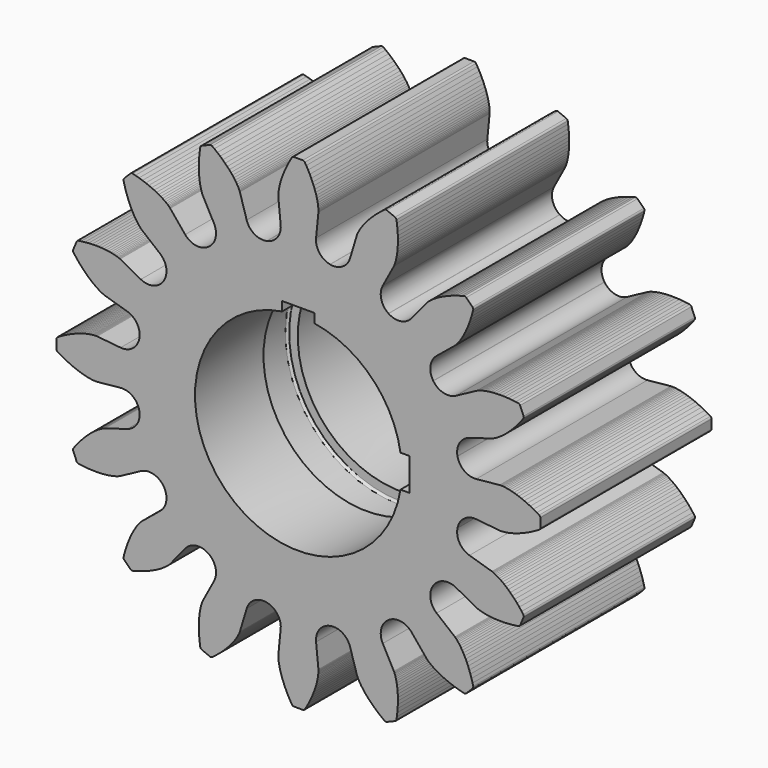
from build123d import *

# Parameters (mm, degrees)
F1_DEPTH = 250


# Not quite as in the source:
# - ends of sketch curves that miss each other by under 0.0002 mm in the source are joined


with BuildPart() as f1:
    # F0 (on Front) → F1 (new body, symmetric)
    with BuildSketch(Plane.XZ):
        with BuildLine():
            ThreePointArc((-371.6747003159, 73.6954086729), (-387.2563589444, 49.0779324218), (-415.3399148314, 41.3240874835))
            Line((-415.3399148314, 41.3240874835), (-470.2256575867, 46.784923388))
            Line((-470.2256575867, 46.784923388), (-471.2844860609, 46.8902713343))
            Line((-471.2844860609, 46.8902713343), (-472.4597318578, 46.9002713343))
            Line((-472.4597318578, 46.9002713343), (-474.0690444775, 46.8465269206))
            Line((-474.0690444775, 46.8465269206), (-476.1124228559, 46.7290391573))
            Line((-476.1124228559, 46.7290391573), (-478.6957490956, 46.5583422005))
            Line((-478.6957490956, 46.5583422005), (-481.6177942115, 46.2074845712))
            Line((-481.6177942115, 46.2074845712), (-485.0797882528, 45.8034166844))
            Line((-485.0797882528, 45.8034166844), (-488.9969184933, 45.1238401788))
            Line((-488.9969184933, 45.1238401788), (-493.252765482, 44.2641030006))
            Line((-493.252765482, 44.2641030006), (-497.963749734, 43.1288550755))
            Line((-497.963749734, 43.1288550755), (-503.1193339008, 41.8239816982))
            Line((-503.1193339008, 41.8239816982), (-508.6347052564, 40.1271813152))
            Line((-508.6347052564, 40.1271813152), (-514.4993296446, 38.1443360289))
            Line((-514.4993296446, 38.1443360289), (-520.8296254522, 35.7800989572))
            Line((-520.8296254522, 35.7800989572), (-527.4032900617, 33.1192817621))
            Line((-527.4032900617, 33.1192817621), (-534.336742924, 30.0665386252))
            Line((-534.336742924, 30.0665386252), (-541.6299829751, 26.6218684827))
            Line((-541.6299829751, 26.6218684827), (-549.1876622686, 22.6688540115))
            Line((-549.1876622686, 22.6688540115), (-556.9992477123, 18.3133773143))
            Line((-556.9992477123, 18.3133773143), (-562.4998031496, 15.0006426899))
            ThreePointArc((-562.4998031496, 15.0006426899), (-564.3868671204, 13.0605402979), (-565.0752713343, 10.4430783145))
            Line((-565.0752713343, 10.4430783145), (-565.0752713343, -10.4430783145))
            ThreePointArc((-565.0752713343, -10.4430783145), (-564.3868671204, -13.0605402979), (-562.4998031027, -15.0006426121))
            Line((-562.4998031027, -15.0006426121), (-556.9992477123, -18.3133773143))
            Line((-556.9992477123, -18.3133773143), (-549.1876622686, -22.6688540115))
            Line((-549.1876622686, -22.6688540115), (-541.6299829751, -26.6218684827))
            Line((-541.6299829751, -26.6218684827), (-534.336742924, -30.0665386252))
            Line((-534.336742924, -30.0665386252), (-527.4032900617, -33.1192817621))
            Line((-527.4032900617, -33.1192817621), (-520.8296254522, -35.7800989572))
            Line((-520.8296254522, -35.7800989572), (-514.4993296446, -38.1443360289))
            Line((-514.4993296446, -38.1443360289), (-508.6347052564, -40.1271813152))
            Line((-508.6347052564, -40.1271813152), (-503.1193339008, -41.8239816982))
            Line((-503.1193339008, -41.8239816982), (-497.963749734, -43.1288550755))
            Line((-497.963749734, -43.1288550755), (-493.252765482, -44.2641030006))
            Line((-493.252765482, -44.2641030006), (-488.9969184933, -45.1238401788))
            Line((-488.9969184933, -45.1238401788), (-485.0797882528, -45.8034166844))
            Line((-485.0797882528, -45.8034166844), (-481.6177942115, -46.2074845712))
            Line((-481.6177942115, -46.2074845712), (-478.6957490956, -46.5583422005))
            Line((-478.6957490956, -46.5583422005), (-476.1124228559, -46.7290391573))
            Line((-476.1124228559, -46.7290391573), (-474.0690444775, -46.8465269206))
            Line((-474.0690444775, -46.8465269206), (-472.4597318578, -46.9002713343))
            Line((-472.4597318578, -46.9002713343), (-471.2844860609, -46.8902713343))
            Line((-471.2844860609, -46.8902713343), (-470.2256575867, -46.784923388))
            Line((-470.2256575867, -46.784923388), (-415.3399148755, -41.3240870398))
            ThreePointArc((-415.3399148755, -41.3240870398), (-387.2563589444, -49.0779324218), (-371.6747003159, -73.6954086729))
            Line((-371.6747003159, -73.6954086729), (-371.5846605661, -74.1480698021))
            ThreePointArc((-371.5846605661, -74.1480698021), (-376.559535795, -102.8544948797), (-399.538090136, -120.7652251933))
            Line((-399.538090136, -120.7652251933), (-452.3356767397, -136.7239348798))
            Line((-452.3356767397, -136.7239348798), (-453.3542211109, -137.0318025112))
            Line((-453.3542211109, -137.0318025112), (-454.4438327304, -137.47231113))
            Line((-454.4438327304, -137.47231113), (-455.910076612, -138.137821877))
            Line((-455.910076612, -138.137821877), (-457.7529516918, -139.028332624))
            Line((-457.7529516918, -139.028332624), (-460.0743115557, -140.1746329006))
            Line((-460.0743115557, -140.1746329006), (-462.6396616301, -141.6170014897))
            Line((-462.6396616301, -141.6170014897), (-465.6834975527, -143.3151585444))
            Line((-465.6834975527, -143.3151585444), (-469.0423909342, -145.442025963))
            Line((-469.0423909342, -145.442025963), (-472.6452734624, -147.864962758))
            Line((-472.6452734624, -147.864962758), (-476.5632145137, -150.716609917))
            Line((-476.5632145137, -150.716609917), (-480.8269993616, -153.89511279))
            Line((-480.8269993616, -153.89511279), (-485.273200681, -157.5733932752))
            Line((-485.273200681, -157.5733932752), (-489.9326058736, -161.6495988508))
            Line((-489.9326058736, -161.6495988508), (-494.8762811236, -166.2563683763))
            Line((-494.8762811236, -166.2563683763), (-499.9313055969, -171.2302745265))
            Line((-499.9313055969, -171.2302745265), (-505.1687465418, -176.703958289))
            Line((-505.1687465418, -176.703958289), (-510.5886039583, -182.6774217919))
            Line((-510.5886039583, -182.6774217919), (-516.0582357949, -189.2217301554))
            Line((-516.0582357949, -189.2217301554), (-521.6084305171, -196.2350297936))
            Line((-521.6084305171, -196.2350297936), (-525.4225526708, -201.400568206))
            ThreePointArc((-525.4225526708, -201.400568206), (-526.4235272395, -203.9151369418), (-526.057870578, -206.5967970892))
            Line((-526.057870578, -206.5967970892), (-518.0650840604, -225.8930910832))
            ThreePointArc((-518.0650840604, -225.8930910832), (-516.4274222611, -228.0478695626), (-513.9415578261, -229.1181424759))
            Line((-513.9415578261, -229.1181424759), (-507.5919780804, -230.0737380294))
            Line((-507.5919780804, -230.0737380294), (-498.7082464354, -231.1083102788))
            Line((-498.7082464354, -231.1083102788), (-490.2131070441, -231.8682208981))
            Line((-490.2131070441, -231.8682208981), (-482.1568142158, -232.259678655))
            Line((-482.1568142158, -232.259678655), (-474.5829048734, -232.4267280272))
            Line((-474.5829048734, -232.4267280272), (-467.4913800809, -232.3693690147))
            Line((-467.4913800809, -232.3693690147), (-460.7381953607, -232.1311406682))
            Line((-460.7381953607, -232.1311406682), (-454.5611864226, -231.7187561183))
            Line((-454.5611864226, -231.7187561183), (-448.8163098532, -231.1757544158))
            Line((-448.8163098532, -231.1757544158), (-443.5538178336, -230.4083432645))
            Line((-443.5538178336, -230.4083432645), (-438.7669961694, -229.6543605022))
            Line((-438.7669961694, -229.6543605022), (-434.506098106, -228.8200117046))
            Line((-434.506098106, -228.8200117046), (-430.6270791658, -227.9488380506))
            Line((-430.6270791658, -227.9488380506), (-427.2739838263, -226.9972994254))
            Line((-427.2739838263, -226.9972994254), (-424.4400989572, -226.2032326027))
            Line((-424.4400989572, -226.2032326027), (-421.9880932113, -225.3723387955))
            Line((-421.9880932113, -225.3723387955), (-420.0552968717, -224.6989167908))
            Line((-420.0552968717, -224.6989167908), (-418.5479197702, -224.1327122792))
            Line((-418.5479197702, -224.1327122792), (-417.4659608427, -223.6737273888))
            Line((-417.4659608427, -223.6737273888), (-416.5280453288, -223.1712023835))
            Line((-416.5280453288, -223.1712023835), (-367.9100031922, -197.1221834433))
            ThreePointArc((-367.9100031922, -197.1221834433), (-338.9969126846, -193.5386902079), (-315.1806367021, -210.3194299305))
            Line((-315.1806367021, -210.3194299305), (-314.924224303, -210.7031772718))
            ThreePointArc((-314.924224303, -210.7031772718), (-308.5349362514, -239.1282583902), (-322.9102125402, -264.4691278049))
            Line((-322.9102125402, -264.4691278049), (-365.5816886572, -299.4178144286))
            Line((-365.5816886572, -299.4178144286), (-366.4048850819, -300.092027027))
            Line((-366.4048850819, -300.092027027), (-367.2429804214, -300.9159810598))
            Line((-367.2429804214, -300.9159810598), (-368.3429325388, -302.0919387104))
            Line((-368.3429325388, -302.0919387104), (-369.7047424984, -303.6199021068))
            Line((-369.7047424984, -303.6199021068), (-371.4107299425, -305.567290913))
            Line((-371.4107299425, -305.567290913), (-373.2288337944, -307.8815833156))
            Line((-373.2288337944, -307.8815833156), (-375.3911151309, -310.6153011279))
            Line((-375.3911151309, -310.6153011279), (-377.6804107257, -313.865662907))
            Line((-377.6804107257, -313.865662907), (-380.0818227282, -317.4829282826))
            Line((-380.0818227282, -317.4829282826), (-382.6102500532, -321.616837625))
            Line((-382.6102500532, -321.616837625), (-385.3331134284, -326.1850712918))
            Line((-385.3331134284, -326.1850712918), (-388.0332506916, -331.28484784))
            Line((-388.0332506916, -331.28484784), (-390.7780836348, -336.8338465631))
            Line((-390.7780836348, -336.8338465631), (-393.5825101085, -342.9818099596))
            Line((-393.5825101085, -342.9818099596), (-396.3493115557, -349.5115737391))
            Line((-396.3493115557, -349.5115737391), (-399.0933879549, -356.5728804001))
            Line((-399.0933879549, -356.5728804001), (-401.8147382422, -364.1657299425))
            Line((-401.8147382422, -364.1657299425), (-404.3636209832, -372.3050202171))
            Line((-404.3636209832, -372.3050202171), (-406.8074579698, -380.9084315812))
            Line((-406.8074579698, -380.9084315812), (-408.3544818046, -387.1403692275))
            ThreePointArc((-408.3544818046, -387.1403692275), (-408.316978103, -389.8465841018), (-406.9529287145, -392.1841843008))
            Line((-406.9529287145, -392.1841843008), (-392.1841838689, -406.9529282826))
            ThreePointArc((-392.1841838689, -406.9529282826), (-389.8465841018, -408.316978103), (-387.140369236, -408.3544817703))
            Line((-387.140369236, -408.3544817703), (-380.9084315812, -406.8074579698))
            Line((-380.9084315812, -406.8074579698), (-372.3050202171, -404.3636209832))
            Line((-372.3050202171, -404.3636209832), (-364.1657299425, -401.8147382422))
            Line((-364.1657299425, -401.8147382422), (-356.5728804001, -399.0933879549))
            Line((-356.5728804001, -399.0933879549), (-349.5115737391, -396.3493115557))
            Line((-349.5115737391, -396.3493115557), (-342.9818099596, -393.5825101085))
            Line((-342.9818099596, -393.5825101085), (-336.8338465631, -390.7780836348))
            Line((-336.8338465631, -390.7780836348), (-331.28484784, -388.0332506916))
            Line((-331.28484784, -388.0332506916), (-326.1850712918, -385.3331134284))
            Line((-326.1850712918, -385.3331134284), (-321.616837625, -382.6102500532))
            Line((-321.616837625, -382.6102500532), (-317.4829282826, -380.0818227282))
            Line((-317.4829282826, -380.0818227282), (-313.865662907, -377.6804107257))
            Line((-313.865662907, -377.6804107257), (-310.6153011279, -375.3911151309))
            Line((-310.6153011279, -375.3911151309), (-307.8815833156, -373.2288337944))
            Line((-307.8815833156, -373.2288337944), (-305.567290913, -371.4107299425))
            Line((-305.567290913, -371.4107299425), (-303.6199021068, -369.7047424984))
            Line((-303.6199021068, -369.7047424984), (-302.0919387104, -368.3429325388))
            Line((-302.0919387104, -368.3429325388), (-300.9159810598, -367.2429804214))
            Line((-300.9159810598, -367.2429804214), (-300.092027027, -366.4048850819))
            Line((-300.092027027, -366.4048850819), (-299.4178144286, -365.5816886572))
            Line((-299.4178144286, -365.5816886572), (-264.4691274739, -322.9102128112))
            ThreePointArc((-264.4691274739, -322.9102128112), (-239.1282583902, -308.5349362514), (-210.7031774657, -314.924224593))
            Line((-210.7031774657, -314.924224593), (-210.3194296659, -315.1806363056))
            ThreePointArc((-210.3194296659, -315.1806363056), (-193.5386902079, -338.9969126846), (-197.1221834078, -367.9100032112))
            Line((-197.1221834078, -367.9100032112), (-223.1712023835, -416.5280453288))
            Line((-223.1712023835, -416.5280453288), (-223.6737273888, -417.4659608427))
            Line((-223.6737273888, -417.4659608427), (-224.1327122792, -418.5479197702))
            Line((-224.1327122792, -418.5479197702), (-224.6989167908, -420.0552968717))
            Line((-224.6989167908, -420.0552968717), (-225.3723387955, -421.9880932113))
            Line((-225.3723387955, -421.9880932113), (-226.2032326027, -424.4400989572))
            Line((-226.2032326027, -424.4400989572), (-226.9972994254, -427.2739838263))
            Line((-226.9972994254, -427.2739838263), (-227.9488380506, -430.6270791658))
            Line((-227.9488380506, -430.6270791658), (-228.8200117046, -434.506098106))
            Line((-228.8200117046, -434.506098106), (-229.6543605022, -438.7669961694))
            Line((-229.6543605022, -438.7669961694), (-230.4083432645, -443.5538178336))
            Line((-230.4083432645, -443.5538178336), (-231.1757544158, -448.8163098532))
            Line((-231.1757544158, -448.8163098532), (-231.7187561183, -454.5611864226))
            Line((-231.7187561183, -454.5611864226), (-232.1311406682, -460.7381953607))
            Line((-232.1311406682, -460.7381953607), (-232.3693690147, -467.4913800809))
            Line((-232.3693690147, -467.4913800809), (-232.4267280272, -474.5829048734))
            Line((-232.4267280272, -474.5829048734), (-232.259678655, -482.1568142158))
            Line((-232.259678655, -482.1568142158), (-231.8682208981, -490.2131070441))
            Line((-231.8682208981, -490.2131070441), (-231.1083102788, -498.7082464354))
            Line((-231.1083102788, -498.7082464354), (-230.0737380294, -507.5919780804))
            Line((-230.0737380294, -507.5919780804), (-229.1181421579, -513.9415577783))
            ThreePointArc((-229.1181421579, -513.9415577783), (-228.0478695626, -516.4274222611), (-225.8930909815, -518.0650838148))
            Line((-225.8930909815, -518.0650838148), (-206.5967971909, -526.0578708236))
            ThreePointArc((-206.5967971909, -526.0578708236), (-203.9151369418, -526.4235272395), (-201.4005682383, -525.4225526271))
            Line((-201.4005682383, -525.4225526271), (-196.2350297936, -521.6084305171))
            Line((-196.2350297936, -521.6084305171), (-189.2217301554, -516.0582357949))
            Line((-189.2217301554, -516.0582357949), (-182.6774217919, -510.5886039583))
            Line((-182.6774217919, -510.5886039583), (-176.703958289, -505.1687465418))
            Line((-176.703958289, -505.1687465418), (-171.2302745265, -499.9313055969))
            Line((-171.2302745265, -499.9313055969), (-166.2563683763, -494.8762811236))
            Line((-166.2563683763, -494.8762811236), (-161.6495988508, -489.9326058736))
            Line((-161.6495988508, -489.9326058736), (-157.5733932752, -485.273200681))
            Line((-157.5733932752, -485.273200681), (-153.89511279, -480.8269993616))
            Line((-153.89511279, -480.8269993616), (-150.716609917, -476.5632145137))
            Line((-150.716609917, -476.5632145137), (-147.864962758, -472.6452734624))
            Line((-147.864962758, -472.6452734624), (-145.442025963, -469.0423909342))
            Line((-145.442025963, -469.0423909342), (-143.3151585444, -465.6834975527))
            Line((-143.3151585444, -465.6834975527), (-141.6170014897, -462.6396616301))
            Line((-141.6170014897, -462.6396616301), (-140.1746329006, -460.0743115557))
            Line((-140.1746329006, -460.0743115557), (-139.028332624, -457.7529516918))
            Line((-139.028332624, -457.7529516918), (-138.137821877, -455.910076612))
            Line((-138.137821877, -455.910076612), (-137.47231113, -454.4438327304))
            Line((-137.47231113, -454.4438327304), (-137.0318025112, -453.3542211109))
            Line((-137.0318025112, -453.3542211109), (-136.7239348798, -452.3356767397))
            Line((-136.7239348798, -452.3356767397), (-120.7652255799, -399.5380900192))
            ThreePointArc((-120.7652255799, -399.5380900192), (-102.8544948797, -376.559535795), (-74.1480698423, -371.5846607676))
            Line((-74.1480698423, -371.5846607676), (-73.6954085976, -371.6746999362))
            ThreePointArc((-73.6954085976, -371.6746999362), (-49.0779324218, -387.2563589444), (-41.3240874835, -415.3399148314))
            Line((-41.3240874835, -415.3399148314), (-46.784923388, -470.2256575867))
            Line((-46.784923388, -470.2256575867), (-46.8902713343, -471.2844860609))
            Line((-46.8902713343, -471.2844860609), (-46.9002713343, -472.4597318578))
            Line((-46.9002713343, -472.4597318578), (-46.8465269206, -474.0690444775))
            Line((-46.8465269206, -474.0690444775), (-46.7290391573, -476.1124228559))
            Line((-46.7290391573, -476.1124228559), (-46.5583422005, -478.6957490956))
            Line((-46.5583422005, -478.6957490956), (-46.2074845712, -481.6177942115))
            Line((-46.2074845712, -481.6177942115), (-45.8034166844, -485.0797882528))
            Line((-45.8034166844, -485.0797882528), (-45.1238401788, -488.9969184933))
            Line((-45.1238401788, -488.9969184933), (-44.2641030006, -493.252765482))
            Line((-44.2641030006, -493.252765482), (-43.1288550755, -497.963749734))
            Line((-43.1288550755, -497.963749734), (-41.8239816982, -503.1193339008))
            Line((-41.8239816982, -503.1193339008), (-40.1271813152, -508.6347052564))
            Line((-40.1271813152, -508.6347052564), (-38.1443360289, -514.4993296446))
            Line((-38.1443360289, -514.4993296446), (-35.7800989572, -520.8296254522))
            Line((-35.7800989572, -520.8296254522), (-33.1192817621, -527.4032900617))
            Line((-33.1192817621, -527.4032900617), (-30.0665386252, -534.336742924))
            Line((-30.0665386252, -534.336742924), (-26.6218684827, -541.6299829751))
            Line((-26.6218684827, -541.6299829751), (-22.6688540115, -549.1876622686))
            Line((-22.6688540115, -549.1876622686), (-18.3133773143, -556.9992477123))
            Line((-18.3133773143, -556.9992477123), (-15.0006426899, -562.4998031496))
            ThreePointArc((-15.0006426899, -562.4998031496), (-13.0605402979, -564.3868671204), (-10.4430783145, -565.0752713343))
            Line((-10.4430783145, -565.0752713343), (10.4430783145, -565.0752713343))
            ThreePointArc((10.4430783145, -565.0752713343), (13.0605402979, -564.3868671204), (15.0006426121, -562.4998031027))
            Line((15.0006426121, -562.4998031027), (18.3133773143, -556.9992477123))
            Line((18.3133773143, -556.9992477123), (22.6688540115, -549.1876622686))
            Line((22.6688540115, -549.1876622686), (26.6218684827, -541.6299829751))
            Line((26.6218684827, -541.6299829751), (30.0665386252, -534.336742924))
            Line((30.0665386252, -534.336742924), (33.1192817621, -527.4032900617))
            Line((33.1192817621, -527.4032900617), (35.7800989572, -520.8296254522))
            Line((35.7800989572, -520.8296254522), (38.1443360289, -514.4993296446))
            Line((38.1443360289, -514.4993296446), (40.1271813152, -508.6347052564))
            Line((40.1271813152, -508.6347052564), (41.8239816982, -503.1193339008))
            Line((41.8239816982, -503.1193339008), (43.1288550755, -497.963749734))
            Line((43.1288550755, -497.963749734), (44.2641030006, -493.252765482))
            Line((44.2641030006, -493.252765482), (45.1238401788, -488.9969184933))
            Line((45.1238401788, -488.9969184933), (45.8034166844, -485.0797882528))
            Line((45.8034166844, -485.0797882528), (46.2074845712, -481.6177942115))
            Line((46.2074845712, -481.6177942115), (46.5583422005, -478.6957490956))
            Line((46.5583422005, -478.6957490956), (46.7290391573, -476.1124228559))
            Line((46.7290391573, -476.1124228559), (46.8465269206, -474.0690444775))
            Line((46.8465269206, -474.0690444775), (46.9002713343, -472.4597318578))
            Line((46.9002713343, -472.4597318578), (46.8902713343, -471.2844860609))
            Line((46.8902713343, -471.2844860609), (46.784923388, -470.2256575867))
            Line((46.784923388, -470.2256575867), (41.3240870398, -415.3399148755))
            ThreePointArc((41.3240870398, -415.3399148755), (49.0779324218, -387.2563589444), (73.6954086729, -371.6747003159))
            Line((73.6954086729, -371.6747003159), (74.1480698021, -371.5846605661))
            ThreePointArc((74.1480698021, -371.5846605661), (102.8544948797, -376.559535795), (120.7652251933, -399.538090136))
            Line((120.7652251933, -399.538090136), (136.7239348798, -452.3356767397))
            Line((136.7239348798, -452.3356767397), (137.0318025112, -453.3542211109))
            Line((137.0318025112, -453.3542211109), (137.47231113, -454.4438327304))
            Line((137.47231113, -454.4438327304), (138.137821877, -455.910076612))
            Line((138.137821877, -455.910076612), (139.028332624, -457.7529516918))
            Line((139.028332624, -457.7529516918), (140.1746329006, -460.0743115557))
            Line((140.1746329006, -460.0743115557), (141.6170014897, -462.6396616301))
            Line((141.6170014897, -462.6396616301), (143.3151585444, -465.6834975527))
            Line((143.3151585444, -465.6834975527), (145.442025963, -469.0423909342))
            Line((145.442025963, -469.0423909342), (147.864962758, -472.6452734624))
            Line((147.864962758, -472.6452734624), (150.716609917, -476.5632145137))
            Line((150.716609917, -476.5632145137), (153.89511279, -480.8269993616))
            Line((153.89511279, -480.8269993616), (157.5733932752, -485.273200681))
            Line((157.5733932752, -485.273200681), (161.6495988508, -489.9326058736))
            Line((161.6495988508, -489.9326058736), (166.2563683763, -494.8762811236))
            Line((166.2563683763, -494.8762811236), (171.2302745265, -499.9313055969))
            Line((171.2302745265, -499.9313055969), (176.703958289, -505.1687465418))
            Line((176.703958289, -505.1687465418), (182.6774217919, -510.5886039583))
            Line((182.6774217919, -510.5886039583), (189.2217301554, -516.0582357949))
            Line((189.2217301554, -516.0582357949), (196.2350297936, -521.6084305171))
            Line((196.2350297936, -521.6084305171), (201.400568206, -525.4225526708))
            ThreePointArc((201.400568206, -525.4225526708), (203.9151369418, -526.4235272395), (206.5967970892, -526.057870578))
            Line((206.5967970892, -526.057870578), (225.8930910832, -518.0650840604))
            ThreePointArc((225.8930910832, -518.0650840604), (228.0478695626, -516.4274222611), (229.1181424759, -513.9415578261))
            Line((229.1181424759, -513.9415578261), (230.0737380294, -507.5919780804))
            Line((230.0737380294, -507.5919780804), (231.1083102788, -498.7082464354))
            Line((231.1083102788, -498.7082464354), (231.8682208981, -490.2131070441))
            Line((231.8682208981, -490.2131070441), (232.259678655, -482.1568142158))
            Line((232.259678655, -482.1568142158), (232.4267280272, -474.5829048734))
            Line((232.4267280272, -474.5829048734), (232.3693690147, -467.4913800809))
            Line((232.3693690147, -467.4913800809), (232.1311406682, -460.7381953607))
            Line((232.1311406682, -460.7381953607), (231.7187561183, -454.5611864226))
            Line((231.7187561183, -454.5611864226), (231.1757544158, -448.8163098532))
            Line((231.1757544158, -448.8163098532), (230.4083432645, -443.5538178336))
            Line((230.4083432645, -443.5538178336), (229.6543605022, -438.7669961694))
            Line((229.6543605022, -438.7669961694), (228.8200117046, -434.506098106))
            Line((228.8200117046, -434.506098106), (227.9488380506, -430.6270791658))
            Line((227.9488380506, -430.6270791658), (226.9972994254, -427.2739838263))
            Line((226.9972994254, -427.2739838263), (226.2032326027, -424.4400989572))
            Line((226.2032326027, -424.4400989572), (225.3723387955, -421.9880932113))
            Line((225.3723387955, -421.9880932113), (224.6989167908, -420.0552968717))
            Line((224.6989167908, -420.0552968717), (224.1327122792, -418.5479197702))
            Line((224.1327122792, -418.5479197702), (223.6737273888, -417.4659608427))
            Line((223.6737273888, -417.4659608427), (223.1712023835, -416.5280453288))
            Line((223.1712023835, -416.5280453288), (197.1221834433, -367.9100031922))
            ThreePointArc((197.1221834433, -367.9100031922), (193.5386902079, -338.9969126846), (210.3194299305, -315.1806367021))
            Line((210.3194299305, -315.1806367021), (210.7031772718, -314.924224303))
            ThreePointArc((210.7031772718, -314.924224303), (239.1282583902, -308.5349362514), (264.4691278049, -322.9102125402))
            Line((264.4691278049, -322.9102125402), (299.4178144286, -365.5816886572))
            Line((299.4178144286, -365.5816886572), (300.092027027, -366.4048850819))
            Line((300.092027027, -366.4048850819), (300.9159810598, -367.2429804214))
            Line((300.9159810598, -367.2429804214), (302.0919387104, -368.3429325388))
            Line((302.0919387104, -368.3429325388), (303.6199021068, -369.7047424984))
            Line((303.6199021068, -369.7047424984), (305.567290913, -371.4107299425))
            Line((305.567290913, -371.4107299425), (307.8815833156, -373.2288337944))
            Line((307.8815833156, -373.2288337944), (310.6153011279, -375.3911151309))
            Line((310.6153011279, -375.3911151309), (313.865662907, -377.6804107257))
            Line((313.865662907, -377.6804107257), (317.4829282826, -380.0818227282))
            Line((317.4829282826, -380.0818227282), (321.616837625, -382.6102500532))
            Line((321.616837625, -382.6102500532), (326.1850712918, -385.3331134284))
            Line((326.1850712918, -385.3331134284), (331.28484784, -388.0332506916))
            Line((331.28484784, -388.0332506916), (336.8338465631, -390.7780836348))
            Line((336.8338465631, -390.7780836348), (342.9818099596, -393.5825101085))
            Line((342.9818099596, -393.5825101085), (349.5115737391, -396.3493115557))
            Line((349.5115737391, -396.3493115557), (356.5728804001, -399.0933879549))
            Line((356.5728804001, -399.0933879549), (364.1657299425, -401.8147382422))
            Line((364.1657299425, -401.8147382422), (372.3050202171, -404.3636209832))
            Line((372.3050202171, -404.3636209832), (380.9084315812, -406.8074579698))
            Line((380.9084315812, -406.8074579698), (387.1403692275, -408.3544818046))
            ThreePointArc((387.1403692275, -408.3544818046), (389.8465841018, -408.316978103), (392.1841843008, -406.9529287145))
            Line((392.1841843008, -406.9529287145), (406.9529282826, -392.1841838689))
            ThreePointArc((406.9529282826, -392.1841838689), (408.316978103, -389.8465841018), (408.3544817703, -387.140369236))
            Line((408.3544817703, -387.140369236), (406.8074579698, -380.9084315812))
            Line((406.8074579698, -380.9084315812), (404.3636209832, -372.3050202171))
            Line((404.3636209832, -372.3050202171), (401.8147382422, -364.1657299425))
            Line((401.8147382422, -364.1657299425), (399.0933879549, -356.5728804001))
            Line((399.0933879549, -356.5728804001), (396.3493115557, -349.5115737391))
            Line((396.3493115557, -349.5115737391), (393.5825101085, -342.9818099596))
            Line((393.5825101085, -342.9818099596), (390.7780836348, -336.8338465631))
            Line((390.7780836348, -336.8338465631), (388.0332506916, -331.28484784))
            Line((388.0332506916, -331.28484784), (385.3331134284, -326.1850712918))
            Line((385.3331134284, -326.1850712918), (382.6102500532, -321.616837625))
            Line((382.6102500532, -321.616837625), (380.0818227282, -317.4829282826))
            Line((380.0818227282, -317.4829282826), (377.6804107257, -313.865662907))
            Line((377.6804107257, -313.865662907), (375.3911151309, -310.6153011279))
            Line((375.3911151309, -310.6153011279), (373.2288337944, -307.8815833156))
            Line((373.2288337944, -307.8815833156), (371.4107299425, -305.567290913))
            Line((371.4107299425, -305.567290913), (369.7047424984, -303.6199021068))
            Line((369.7047424984, -303.6199021068), (368.3429325388, -302.0919387104))
            Line((368.3429325388, -302.0919387104), (367.2429804214, -300.9159810598))
            Line((367.2429804214, -300.9159810598), (366.4048850819, -300.092027027))
            Line((366.4048850819, -300.092027027), (365.5816886572, -299.4178144286))
            Line((365.5816886572, -299.4178144286), (322.9102128112, -264.4691274739))
            ThreePointArc((322.9102128112, -264.4691274739), (308.5349362514, -239.1282583902), (314.924224593, -210.7031774657))
            Line((314.924224593, -210.7031774657), (315.1806363056, -210.3194296659))
            ThreePointArc((315.1806363056, -210.3194296659), (338.9969126846, -193.5386902079), (367.9100032112, -197.1221834078))
            Line((367.9100032112, -197.1221834078), (416.5280453288, -223.1712023835))
            Line((416.5280453288, -223.1712023835), (417.4659608427, -223.6737273888))
            Line((417.4659608427, -223.6737273888), (418.5479197702, -224.1327122792))
            Line((418.5479197702, -224.1327122792), (420.0552968717, -224.6989167908))
            Line((420.0552968717, -224.6989167908), (421.9880932113, -225.3723387955))
            Line((421.9880932113, -225.3723387955), (424.4400989572, -226.2032326027))
            Line((424.4400989572, -226.2032326027), (427.2739838263, -226.9972994254))
            Line((427.2739838263, -226.9972994254), (430.6270791658, -227.9488380506))
            Line((430.6270791658, -227.9488380506), (434.506098106, -228.8200117046))
            Line((434.506098106, -228.8200117046), (438.7669961694, -229.6543605022))
            Line((438.7669961694, -229.6543605022), (443.5538178336, -230.4083432645))
            Line((443.5538178336, -230.4083432645), (448.8163098532, -231.1757544158))
            Line((448.8163098532, -231.1757544158), (454.5611864226, -231.7187561183))
            Line((454.5611864226, -231.7187561183), (460.7381953607, -232.1311406682))
            Line((460.7381953607, -232.1311406682), (467.4913800809, -232.3693690147))
            Line((467.4913800809, -232.3693690147), (474.5829048734, -232.4267280272))
            Line((474.5829048734, -232.4267280272), (482.1568142158, -232.259678655))
            Line((482.1568142158, -232.259678655), (490.2131070441, -231.8682208981))
            Line((490.2131070441, -231.8682208981), (498.7082464354, -231.1083102788))
            Line((498.7082464354, -231.1083102788), (507.5919780804, -230.0737380294))
            Line((507.5919780804, -230.0737380294), (513.9415577783, -229.1181421579))
            ThreePointArc((513.9415577783, -229.1181421579), (516.4274222611, -228.0478695626), (518.0650838148, -225.8930909815))
            Line((518.0650838148, -225.8930909815), (526.0578708236, -206.5967971909))
            ThreePointArc((526.0578708236, -206.5967971909), (526.4235272395, -203.9151369418), (525.4225526271, -201.4005682383))
            Line((525.4225526271, -201.4005682383), (521.6084305171, -196.2350297936))
            Line((521.6084305171, -196.2350297936), (516.0582357949, -189.2217301554))
            Line((516.0582357949, -189.2217301554), (510.5886039583, -182.6774217919))
            Line((510.5886039583, -182.6774217919), (505.1687465418, -176.703958289))
            Line((505.1687465418, -176.703958289), (499.9313055969, -171.2302745265))
            Line((499.9313055969, -171.2302745265), (494.8762811236, -166.2563683763))
            Line((494.8762811236, -166.2563683763), (489.9326058736, -161.6495988508))
            Line((489.9326058736, -161.6495988508), (485.273200681, -157.5733932752))
            Line((485.273200681, -157.5733932752), (480.8269993616, -153.89511279))
            Line((480.8269993616, -153.89511279), (476.5632145137, -150.716609917))
            Line((476.5632145137, -150.716609917), (472.6452734624, -147.864962758))
            Line((472.6452734624, -147.864962758), (469.0423909342, -145.442025963))
            Line((469.0423909342, -145.442025963), (465.6834975527, -143.3151585444))
            Line((465.6834975527, -143.3151585444), (462.6396616301, -141.6170014897))
            Line((462.6396616301, -141.6170014897), (460.0743115557, -140.1746329006))
            Line((460.0743115557, -140.1746329006), (457.7529516918, -139.028332624))
            Line((457.7529516918, -139.028332624), (455.910076612, -138.137821877))
            Line((455.910076612, -138.137821877), (454.4438327304, -137.47231113))
            Line((454.4438327304, -137.47231113), (453.3542211109, -137.0318025112))
            Line((453.3542211109, -137.0318025112), (452.3356767397, -136.7239348798))
            Line((452.3356767397, -136.7239348798), (399.5380900192, -120.7652255799))
            ThreePointArc((399.5380900192, -120.7652255799), (376.559535795, -102.8544948797), (371.5846607676, -74.1480698423))
            Line((371.5846607676, -74.1480698423), (371.6746999362, -73.6954085976))
            ThreePointArc((371.6746999362, -73.6954085976), (387.2563589444, -49.0779324218), (415.3399148314, -41.3240874835))
            Line((415.3399148314, -41.3240874835), (470.2256575867, -46.784923388))
            Line((470.2256575867, -46.784923388), (471.2844860609, -46.8902713343))
            Line((471.2844860609, -46.8902713343), (472.4597318578, -46.9002713343))
            Line((472.4597318578, -46.9002713343), (474.0690444775, -46.8465269206))
            Line((474.0690444775, -46.8465269206), (476.1124228559, -46.7290391573))
            Line((476.1124228559, -46.7290391573), (478.6957490956, -46.5583422005))
            Line((478.6957490956, -46.5583422005), (481.6177942115, -46.2074845712))
            Line((481.6177942115, -46.2074845712), (485.0797882528, -45.8034166844))
            Line((485.0797882528, -45.8034166844), (488.9969184933, -45.1238401788))
            Line((488.9969184933, -45.1238401788), (493.252765482, -44.2641030006))
            Line((493.252765482, -44.2641030006), (497.963749734, -43.1288550755))
            Line((497.963749734, -43.1288550755), (503.1193339008, -41.8239816982))
            Line((503.1193339008, -41.8239816982), (508.6347052564, -40.1271813152))
            Line((508.6347052564, -40.1271813152), (514.4993296446, -38.1443360289))
            Line((514.4993296446, -38.1443360289), (520.8296254522, -35.7800989572))
            Line((520.8296254522, -35.7800989572), (527.4032900617, -33.1192817621))
            Line((527.4032900617, -33.1192817621), (534.336742924, -30.0665386252))
            Line((534.336742924, -30.0665386252), (541.6299829751, -26.6218684827))
            Line((541.6299829751, -26.6218684827), (549.1876622686, -22.6688540115))
            Line((549.1876622686, -22.6688540115), (556.9992477123, -18.3133773143))
            Line((556.9992477123, -18.3133773143), (562.4998031496, -15.0006426899))
            ThreePointArc((562.4998031496, -15.0006426899), (564.3868671204, -13.0605402979), (565.0752713343, -10.4430783145))
            Line((565.0752713343, -10.4430783145), (565.0752713343, 10.4430783145))
            ThreePointArc((565.0752713343, 10.4430783145), (564.3868671204, 13.0605402979), (562.4998031027, 15.0006426121))
            Line((562.4998031027, 15.0006426121), (556.9992477123, 18.3133773143))
            Line((556.9992477123, 18.3133773143), (549.1876622686, 22.6688540115))
            Line((549.1876622686, 22.6688540115), (541.6299829751, 26.6218684827))
            Line((541.6299829751, 26.6218684827), (534.336742924, 30.0665386252))
            Line((534.336742924, 30.0665386252), (527.4032900617, 33.1192817621))
            Line((527.4032900617, 33.1192817621), (520.8296254522, 35.7800989572))
            Line((520.8296254522, 35.7800989572), (514.4993296446, 38.1443360289))
            Line((514.4993296446, 38.1443360289), (508.6347052564, 40.1271813152))
            Line((508.6347052564, 40.1271813152), (503.1193339008, 41.8239816982))
            Line((503.1193339008, 41.8239816982), (497.963749734, 43.1288550755))
            Line((497.963749734, 43.1288550755), (493.252765482, 44.2641030006))
            Line((493.252765482, 44.2641030006), (488.9969184933, 45.1238401788))
            Line((488.9969184933, 45.1238401788), (485.0797882528, 45.8034166844))
            Line((485.0797882528, 45.8034166844), (481.6177942115, 46.2074845712))
            Line((481.6177942115, 46.2074845712), (478.6957490956, 46.5583422005))
            Line((478.6957490956, 46.5583422005), (476.1124228559, 46.7290391573))
            Line((476.1124228559, 46.7290391573), (474.0690444775, 46.8465269206))
            Line((474.0690444775, 46.8465269206), (472.4597318578, 46.9002713343))
            Line((472.4597318578, 46.9002713343), (471.2844860609, 46.8902713343))
            Line((471.2844860609, 46.8902713343), (470.2256575867, 46.784923388))
            Line((470.2256575867, 46.784923388), (415.3399148755, 41.3240870398))
            ThreePointArc((415.3399148755, 41.3240870398), (387.2563589444, 49.0779324218), (371.6747003159, 73.6954086729))
            Line((371.6747003159, 73.6954086729), (371.5846605661, 74.1480698021))
            ThreePointArc((371.5846605661, 74.1480698021), (376.559535795, 102.8544948797), (399.538090136, 120.7652251933))
            Line((399.538090136, 120.7652251933), (452.3356767397, 136.7239348798))
            Line((452.3356767397, 136.7239348798), (453.3542211109, 137.0318025112))
            Line((453.3542211109, 137.0318025112), (454.4438327304, 137.47231113))
            Line((454.4438327304, 137.47231113), (455.910076612, 138.137821877))
            Line((455.910076612, 138.137821877), (457.7529516918, 139.028332624))
            Line((457.7529516918, 139.028332624), (460.0743115557, 140.1746329006))
            Line((460.0743115557, 140.1746329006), (462.6396616301, 141.6170014897))
            Line((462.6396616301, 141.6170014897), (465.6834975527, 143.3151585444))
            Line((465.6834975527, 143.3151585444), (469.0423909342, 145.442025963))
            Line((469.0423909342, 145.442025963), (472.6452734624, 147.864962758))
            Line((472.6452734624, 147.864962758), (476.5632145137, 150.716609917))
            Line((476.5632145137, 150.716609917), (480.8269993616, 153.89511279))
            Line((480.8269993616, 153.89511279), (485.273200681, 157.5733932752))
            Line((485.273200681, 157.5733932752), (489.9326058736, 161.6495988508))
            Line((489.9326058736, 161.6495988508), (494.8762811236, 166.2563683763))
            Line((494.8762811236, 166.2563683763), (499.9313055969, 171.2302745265))
            Line((499.9313055969, 171.2302745265), (505.1687465418, 176.703958289))
            Line((505.1687465418, 176.703958289), (510.5886039583, 182.6774217919))
            Line((510.5886039583, 182.6774217919), (516.0582357949, 189.2217301554))
            Line((516.0582357949, 189.2217301554), (521.6084305171, 196.2350297936))
            Line((521.6084305171, 196.2350297936), (525.4225526708, 201.400568206))
            ThreePointArc((525.4225526708, 201.400568206), (526.4235272395, 203.9151369418), (526.057870578, 206.5967970892))
            Line((526.057870578, 206.5967970892), (518.0650840604, 225.8930910832))
            ThreePointArc((518.0650840604, 225.8930910832), (516.4274222611, 228.0478695626), (513.9415578261, 229.1181424759))
            Line((513.9415578261, 229.1181424759), (507.5919780804, 230.0737380294))
            Line((507.5919780804, 230.0737380294), (498.7082464354, 231.1083102788))
            Line((498.7082464354, 231.1083102788), (490.2131070441, 231.8682208981))
            Line((490.2131070441, 231.8682208981), (482.1568142158, 232.259678655))
            Line((482.1568142158, 232.259678655), (474.5829048734, 232.4267280272))
            Line((474.5829048734, 232.4267280272), (467.4913800809, 232.3693690147))
            Line((467.4913800809, 232.3693690147), (460.7381953607, 232.1311406682))
            Line((460.7381953607, 232.1311406682), (454.5611864226, 231.7187561183))
            Line((454.5611864226, 231.7187561183), (448.8163098532, 231.1757544158))
            Line((448.8163098532, 231.1757544158), (443.5538178336, 230.4083432645))
            Line((443.5538178336, 230.4083432645), (438.7669961694, 229.6543605022))
            Line((438.7669961694, 229.6543605022), (434.506098106, 228.8200117046))
            Line((434.506098106, 228.8200117046), (430.6270791658, 227.9488380506))
            Line((430.6270791658, 227.9488380506), (427.2739838263, 226.9972994254))
            Line((427.2739838263, 226.9972994254), (424.4400989572, 226.2032326027))
            Line((424.4400989572, 226.2032326027), (421.9880932113, 225.3723387955))
            Line((421.9880932113, 225.3723387955), (420.0552968717, 224.6989167908))
            Line((420.0552968717, 224.6989167908), (418.5479197702, 224.1327122792))
            Line((418.5479197702, 224.1327122792), (417.4659608427, 223.6737273888))
            Line((417.4659608427, 223.6737273888), (416.5280453288, 223.1712023835))
            Line((416.5280453288, 223.1712023835), (367.9100031922, 197.1221834433))
            ThreePointArc((367.9100031922, 197.1221834433), (338.9969126846, 193.5386902079), (315.1806367021, 210.3194299305))
            Line((315.1806367021, 210.3194299305), (314.924224303, 210.7031772718))
            ThreePointArc((314.924224303, 210.7031772718), (308.5349362514, 239.1282583902), (322.9102125402, 264.4691278049))
            Line((322.9102125402, 264.4691278049), (365.5816886572, 299.4178144286))
            Line((365.5816886572, 299.4178144286), (366.4048850819, 300.092027027))
            Line((366.4048850819, 300.092027027), (367.2429804214, 300.9159810598))
            Line((367.2429804214, 300.9159810598), (368.3429325388, 302.0919387104))
            Line((368.3429325388, 302.0919387104), (369.7047424984, 303.6199021068))
            Line((369.7047424984, 303.6199021068), (371.4107299425, 305.567290913))
            Line((371.4107299425, 305.567290913), (373.2288337944, 307.8815833156))
            Line((373.2288337944, 307.8815833156), (375.3911151309, 310.6153011279))
            Line((375.3911151309, 310.6153011279), (377.6804107257, 313.865662907))
            Line((377.6804107257, 313.865662907), (380.0818227282, 317.4829282826))
            Line((380.0818227282, 317.4829282826), (382.6102500532, 321.616837625))
            Line((382.6102500532, 321.616837625), (385.3331134284, 326.1850712918))
            Line((385.3331134284, 326.1850712918), (388.0332506916, 331.28484784))
            Line((388.0332506916, 331.28484784), (390.7780836348, 336.8338465631))
            Line((390.7780836348, 336.8338465631), (393.5825101085, 342.9818099596))
            Line((393.5825101085, 342.9818099596), (396.3493115557, 349.5115737391))
            Line((396.3493115557, 349.5115737391), (399.0933879549, 356.5728804001))
            Line((399.0933879549, 356.5728804001), (401.8147382422, 364.1657299425))
            Line((401.8147382422, 364.1657299425), (404.3636209832, 372.3050202171))
            Line((404.3636209832, 372.3050202171), (406.8074579698, 380.9084315812))
            Line((406.8074579698, 380.9084315812), (408.3544818046, 387.1403692275))
            ThreePointArc((408.3544818046, 387.1403692275), (408.316978103, 389.8465841018), (406.9529287145, 392.1841843008))
            Line((406.9529287145, 392.1841843008), (392.1841838689, 406.9529282826))
            ThreePointArc((392.1841838689, 406.9529282826), (389.8465841018, 408.316978103), (387.140369236, 408.3544817703))
            Line((387.140369236, 408.3544817703), (380.9084315812, 406.8074579698))
            Line((380.9084315812, 406.8074579698), (372.3050202171, 404.3636209832))
            Line((372.3050202171, 404.3636209832), (364.1657299425, 401.8147382422))
            Line((364.1657299425, 401.8147382422), (356.5728804001, 399.0933879549))
            Line((356.5728804001, 399.0933879549), (349.5115737391, 396.3493115557))
            Line((349.5115737391, 396.3493115557), (342.9818099596, 393.5825101085))
            Line((342.9818099596, 393.5825101085), (336.8338465631, 390.7780836348))
            Line((336.8338465631, 390.7780836348), (331.28484784, 388.0332506916))
            Line((331.28484784, 388.0332506916), (326.1850712918, 385.3331134284))
            Line((326.1850712918, 385.3331134284), (321.616837625, 382.6102500532))
            Line((321.616837625, 382.6102500532), (317.4829282826, 380.0818227282))
            Line((317.4829282826, 380.0818227282), (313.865662907, 377.6804107257))
            Line((313.865662907, 377.6804107257), (310.6153011279, 375.3911151309))
            Line((310.6153011279, 375.3911151309), (307.8815833156, 373.2288337944))
            Line((307.8815833156, 373.2288337944), (305.567290913, 371.4107299425))
            Line((305.567290913, 371.4107299425), (303.6199021068, 369.7047424984))
            Line((303.6199021068, 369.7047424984), (302.0919387104, 368.3429325388))
            Line((302.0919387104, 368.3429325388), (300.9159810598, 367.2429804214))
            Line((300.9159810598, 367.2429804214), (300.092027027, 366.4048850819))
            Line((300.092027027, 366.4048850819), (299.4178144286, 365.5816886572))
            Line((299.4178144286, 365.5816886572), (264.4691274739, 322.9102128112))
            ThreePointArc((264.4691274739, 322.9102128112), (239.1282583902, 308.5349362514), (210.7031774657, 314.924224593))
            Line((210.7031774657, 314.924224593), (210.3194296659, 315.1806363056))
            ThreePointArc((210.3194296659, 315.1806363056), (193.5386902079, 338.9969126846), (197.1221834078, 367.9100032112))
            Line((197.1221834078, 367.9100032112), (223.1712023835, 416.5280453288))
            Line((223.1712023835, 416.5280453288), (223.6737273888, 417.4659608427))
            Line((223.6737273888, 417.4659608427), (224.1327122792, 418.5479197702))
            Line((224.1327122792, 418.5479197702), (224.6989167908, 420.0552968717))
            Line((224.6989167908, 420.0552968717), (225.3723387955, 421.9880932113))
            Line((225.3723387955, 421.9880932113), (226.2032326027, 424.4400989572))
            Line((226.2032326027, 424.4400989572), (226.9972994254, 427.2739838263))
            Line((226.9972994254, 427.2739838263), (227.9488380506, 430.6270791658))
            Line((227.9488380506, 430.6270791658), (228.8200117046, 434.506098106))
            Line((228.8200117046, 434.506098106), (229.6543605022, 438.7669961694))
            Line((229.6543605022, 438.7669961694), (230.4083432645, 443.5538178336))
            Line((230.4083432645, 443.5538178336), (231.1757544158, 448.8163098532))
            Line((231.1757544158, 448.8163098532), (231.7187561183, 454.5611864226))
            Line((231.7187561183, 454.5611864226), (232.1311406682, 460.7381953607))
            Line((232.1311406682, 460.7381953607), (232.3693690147, 467.4913800809))
            Line((232.3693690147, 467.4913800809), (232.4267280272, 474.5829048734))
            Line((232.4267280272, 474.5829048734), (232.259678655, 482.1568142158))
            Line((232.259678655, 482.1568142158), (231.8682208981, 490.2131070441))
            Line((231.8682208981, 490.2131070441), (231.1083102788, 498.7082464354))
            Line((231.1083102788, 498.7082464354), (230.0737380294, 507.5919780804))
            Line((230.0737380294, 507.5919780804), (229.1181421579, 513.9415577783))
            ThreePointArc((229.1181421579, 513.9415577783), (228.0478695626, 516.4274222611), (225.8930909815, 518.0650838148))
            Line((225.8930909815, 518.0650838148), (206.5967971909, 526.0578708236))
            ThreePointArc((206.5967971909, 526.0578708236), (203.9151369418, 526.4235272395), (201.4005682383, 525.4225526271))
            Line((201.4005682383, 525.4225526271), (196.2350297936, 521.6084305171))
            Line((196.2350297936, 521.6084305171), (189.2217301554, 516.0582357949))
            Line((189.2217301554, 516.0582357949), (182.6774217919, 510.5886039583))
            Line((182.6774217919, 510.5886039583), (176.703958289, 505.1687465418))
            Line((176.703958289, 505.1687465418), (171.2302745265, 499.9313055969))
            Line((171.2302745265, 499.9313055969), (166.2563683763, 494.8762811236))
            Line((166.2563683763, 494.8762811236), (161.6495988508, 489.9326058736))
            Line((161.6495988508, 489.9326058736), (157.5733932752, 485.273200681))
            Line((157.5733932752, 485.273200681), (153.89511279, 480.8269993616))
            Line((153.89511279, 480.8269993616), (150.716609917, 476.5632145137))
            Line((150.716609917, 476.5632145137), (147.864962758, 472.6452734624))
            Line((147.864962758, 472.6452734624), (145.442025963, 469.0423909342))
            Line((145.442025963, 469.0423909342), (143.3151585444, 465.6834975527))
            Line((143.3151585444, 465.6834975527), (141.6170014897, 462.6396616301))
            Line((141.6170014897, 462.6396616301), (140.1746329006, 460.0743115557))
            Line((140.1746329006, 460.0743115557), (139.028332624, 457.7529516918))
            Line((139.028332624, 457.7529516918), (138.137821877, 455.910076612))
            Line((138.137821877, 455.910076612), (137.47231113, 454.4438327304))
            Line((137.47231113, 454.4438327304), (137.0318025112, 453.3542211109))
            Line((137.0318025112, 453.3542211109), (136.7239348798, 452.3356767397))
            Line((136.7239348798, 452.3356767397), (120.7652255799, 399.5380900192))
            ThreePointArc((120.7652255799, 399.5380900192), (102.8544948797, 376.559535795), (74.1480698423, 371.5846607676))
            Line((74.1480698423, 371.5846607676), (73.6954085976, 371.6746999362))
            ThreePointArc((73.6954085976, 371.6746999362), (49.0779324218, 387.2563589444), (41.3240874835, 415.3399148314))
            Line((41.3240874835, 415.3399148314), (46.784923388, 470.2256575867))
            Line((46.784923388, 470.2256575867), (46.8902713343, 471.2844860609))
            Line((46.8902713343, 471.2844860609), (46.9002713343, 472.4597318578))
            Line((46.9002713343, 472.4597318578), (46.8465269206, 474.0690444775))
            Line((46.8465269206, 474.0690444775), (46.7290391573, 476.1124228559))
            Line((46.7290391573, 476.1124228559), (46.5583422005, 478.6957490956))
            Line((46.5583422005, 478.6957490956), (46.2074845712, 481.6177942115))
            Line((46.2074845712, 481.6177942115), (45.8034166844, 485.0797882528))
            Line((45.8034166844, 485.0797882528), (45.1238401788, 488.9969184933))
            Line((45.1238401788, 488.9969184933), (44.2641030006, 493.252765482))
            Line((44.2641030006, 493.252765482), (43.1288550755, 497.963749734))
            Line((43.1288550755, 497.963749734), (41.8239816982, 503.1193339008))
            Line((41.8239816982, 503.1193339008), (40.1271813152, 508.6347052564))
            Line((40.1271813152, 508.6347052564), (38.1443360289, 514.4993296446))
            Line((38.1443360289, 514.4993296446), (35.7800989572, 520.8296254522))
            Line((35.7800989572, 520.8296254522), (33.1192817621, 527.4032900617))
            Line((33.1192817621, 527.4032900617), (30.0665386252, 534.336742924))
            Line((30.0665386252, 534.336742924), (26.6218684827, 541.6299829751))
            Line((26.6218684827, 541.6299829751), (22.6688540115, 549.1876622686))
            Line((22.6688540115, 549.1876622686), (18.3133773143, 556.9992477123))
            Line((18.3133773143, 556.9992477123), (15.0006426899, 562.4998031496))
            ThreePointArc((15.0006426899, 562.4998031496), (13.0605402979, 564.3868671204), (10.4430783145, 565.0752713343))
            Line((10.4430783145, 565.0752713343), (-10.4430783145, 565.0752713343))
            ThreePointArc((-10.4430783145, 565.0752713343), (-13.0605402979, 564.3868671204), (-15.0006426121, 562.4998031027))
            Line((-15.0006426121, 562.4998031027), (-18.3133773143, 556.9992477123))
            Line((-18.3133773143, 556.9992477123), (-22.6688540115, 549.1876622686))
            Line((-22.6688540115, 549.1876622686), (-26.6218684827, 541.6299829751))
            Line((-26.6218684827, 541.6299829751), (-30.0665386252, 534.336742924))
            Line((-30.0665386252, 534.336742924), (-33.1192817621, 527.4032900617))
            Line((-33.1192817621, 527.4032900617), (-35.7800989572, 520.8296254522))
            Line((-35.7800989572, 520.8296254522), (-38.1443360289, 514.4993296446))
            Line((-38.1443360289, 514.4993296446), (-40.1271813152, 508.6347052564))
            Line((-40.1271813152, 508.6347052564), (-41.8239816982, 503.1193339008))
            Line((-41.8239816982, 503.1193339008), (-43.1288550755, 497.963749734))
            Line((-43.1288550755, 497.963749734), (-44.2641030006, 493.252765482))
            Line((-44.2641030006, 493.252765482), (-45.1238401788, 488.9969184933))
            Line((-45.1238401788, 488.9969184933), (-45.8034166844, 485.0797882528))
            Line((-45.8034166844, 485.0797882528), (-46.2074845712, 481.6177942115))
            Line((-46.2074845712, 481.6177942115), (-46.5583422005, 478.6957490956))
            Line((-46.5583422005, 478.6957490956), (-46.7290391573, 476.1124228559))
            Line((-46.7290391573, 476.1124228559), (-46.8465269206, 474.0690444775))
            Line((-46.8465269206, 474.0690444775), (-46.9002713343, 472.4597318578))
            Line((-46.9002713343, 472.4597318578), (-46.8902713343, 471.2844860609))
            Line((-46.8902713343, 471.2844860609), (-46.784923388, 470.2256575867))
            Line((-46.784923388, 470.2256575867), (-41.3240870398, 415.3399148755))
            ThreePointArc((-41.3240870398, 415.3399148755), (-49.0779324218, 387.2563589444), (-73.6954086729, 371.6747003159))
            Line((-73.6954086729, 371.6747003159), (-74.1480698021, 371.5846605661))
            ThreePointArc((-74.1480698021, 371.5846605661), (-102.8544948797, 376.559535795), (-120.7652251933, 399.538090136))
            Line((-120.7652251933, 399.538090136), (-136.7239348798, 452.3356767397))
            Line((-136.7239348798, 452.3356767397), (-137.0318025112, 453.3542211109))
            Line((-137.0318025112, 453.3542211109), (-137.47231113, 454.4438327304))
            Line((-137.47231113, 454.4438327304), (-138.137821877, 455.910076612))
            Line((-138.137821877, 455.910076612), (-139.028332624, 457.7529516918))
            Line((-139.028332624, 457.7529516918), (-140.1746329006, 460.0743115557))
            Line((-140.1746329006, 460.0743115557), (-141.6170014897, 462.6396616301))
            Line((-141.6170014897, 462.6396616301), (-143.3151585444, 465.6834975527))
            Line((-143.3151585444, 465.6834975527), (-145.442025963, 469.0423909342))
            Line((-145.442025963, 469.0423909342), (-147.864962758, 472.6452734624))
            Line((-147.864962758, 472.6452734624), (-150.716609917, 476.5632145137))
            Line((-150.716609917, 476.5632145137), (-153.89511279, 480.8269993616))
            Line((-153.89511279, 480.8269993616), (-157.5733932752, 485.273200681))
            Line((-157.5733932752, 485.273200681), (-161.6495988508, 489.9326058736))
            Line((-161.6495988508, 489.9326058736), (-166.2563683763, 494.8762811236))
            Line((-166.2563683763, 494.8762811236), (-171.2302745265, 499.9313055969))
            Line((-171.2302745265, 499.9313055969), (-176.703958289, 505.1687465418))
            Line((-176.703958289, 505.1687465418), (-182.6774217919, 510.5886039583))
            Line((-182.6774217919, 510.5886039583), (-189.2217301554, 516.0582357949))
            Line((-189.2217301554, 516.0582357949), (-196.2350297936, 521.6084305171))
            Line((-196.2350297936, 521.6084305171), (-201.400568206, 525.4225526708))
            ThreePointArc((-201.400568206, 525.4225526708), (-203.9151369418, 526.4235272395), (-206.5967970892, 526.057870578))
            Line((-206.5967970892, 526.057870578), (-225.8930910832, 518.0650840604))
            ThreePointArc((-225.8930910832, 518.0650840604), (-228.0478695626, 516.4274222611), (-229.1181424759, 513.9415578261))
            Line((-229.1181424759, 513.9415578261), (-230.0737380294, 507.5919780804))
            Line((-230.0737380294, 507.5919780804), (-231.1083102788, 498.7082464354))
            Line((-231.1083102788, 498.7082464354), (-231.8682208981, 490.2131070441))
            Line((-231.8682208981, 490.2131070441), (-232.259678655, 482.1568142158))
            Line((-232.259678655, 482.1568142158), (-232.4267280272, 474.5829048734))
            Line((-232.4267280272, 474.5829048734), (-232.3693690147, 467.4913800809))
            Line((-232.3693690147, 467.4913800809), (-232.1311406682, 460.7381953607))
            Line((-232.1311406682, 460.7381953607), (-231.7187561183, 454.5611864226))
            Line((-231.7187561183, 454.5611864226), (-231.1757544158, 448.8163098532))
            Line((-231.1757544158, 448.8163098532), (-230.4083432645, 443.5538178336))
            Line((-230.4083432645, 443.5538178336), (-229.6543605022, 438.7669961694))
            Line((-229.6543605022, 438.7669961694), (-228.8200117046, 434.506098106))
            Line((-228.8200117046, 434.506098106), (-227.9488380506, 430.6270791658))
            Line((-227.9488380506, 430.6270791658), (-226.9972994254, 427.2739838263))
            Line((-226.9972994254, 427.2739838263), (-226.2032326027, 424.4400989572))
            Line((-226.2032326027, 424.4400989572), (-225.3723387955, 421.9880932113))
            Line((-225.3723387955, 421.9880932113), (-224.6989167908, 420.0552968717))
            Line((-224.6989167908, 420.0552968717), (-224.1327122792, 418.5479197702))
            Line((-224.1327122792, 418.5479197702), (-223.6737273888, 417.4659608427))
            Line((-223.6737273888, 417.4659608427), (-223.1712023835, 416.5280453288))
            Line((-223.1712023835, 416.5280453288), (-197.1221834433, 367.9100031922))
            ThreePointArc((-197.1221834433, 367.9100031922), (-193.5386902079, 338.9969126846), (-210.3194299305, 315.1806367021))
            Line((-210.3194299305, 315.1806367021), (-210.7031772718, 314.924224303))
            ThreePointArc((-210.7031772718, 314.924224303), (-239.1282583902, 308.5349362514), (-264.4691278049, 322.9102125402))
            Line((-264.4691278049, 322.9102125402), (-299.4178144286, 365.5816886572))
            Line((-299.4178144286, 365.5816886572), (-300.092027027, 366.4048850819))
            Line((-300.092027027, 366.4048850819), (-300.9159810598, 367.2429804214))
            Line((-300.9159810598, 367.2429804214), (-302.0919387104, 368.3429325388))
            Line((-302.0919387104, 368.3429325388), (-303.6199021068, 369.7047424984))
            Line((-303.6199021068, 369.7047424984), (-305.567290913, 371.4107299425))
            Line((-305.567290913, 371.4107299425), (-307.8815833156, 373.2288337944))
            Line((-307.8815833156, 373.2288337944), (-310.6153011279, 375.3911151309))
            Line((-310.6153011279, 375.3911151309), (-313.865662907, 377.6804107257))
            Line((-313.865662907, 377.6804107257), (-317.4829282826, 380.0818227282))
            Line((-317.4829282826, 380.0818227282), (-321.616837625, 382.6102500532))
            Line((-321.616837625, 382.6102500532), (-326.1850712918, 385.3331134284))
            Line((-326.1850712918, 385.3331134284), (-331.28484784, 388.0332506916))
            Line((-331.28484784, 388.0332506916), (-336.8338465631, 390.7780836348))
            Line((-336.8338465631, 390.7780836348), (-342.9818099596, 393.5825101085))
            Line((-342.9818099596, 393.5825101085), (-349.5115737391, 396.3493115557))
            Line((-349.5115737391, 396.3493115557), (-356.5728804001, 399.0933879549))
            Line((-356.5728804001, 399.0933879549), (-364.1657299425, 401.8147382422))
            Line((-364.1657299425, 401.8147382422), (-372.3050202171, 404.3636209832))
            Line((-372.3050202171, 404.3636209832), (-380.9084315812, 406.8074579698))
            Line((-380.9084315812, 406.8074579698), (-387.1403692275, 408.3544818046))
            ThreePointArc((-387.1403692275, 408.3544818046), (-389.8465841018, 408.316978103), (-392.1841843008, 406.9529287145))
            Line((-392.1841843008, 406.9529287145), (-406.9529282826, 392.1841838689))
            ThreePointArc((-406.9529282826, 392.1841838689), (-408.316978103, 389.8465841018), (-408.3544817703, 387.140369236))
            Line((-408.3544817703, 387.140369236), (-406.8074579698, 380.9084315812))
            Line((-406.8074579698, 380.9084315812), (-404.3636209832, 372.3050202171))
            Line((-404.3636209832, 372.3050202171), (-401.8147382422, 364.1657299425))
            Line((-401.8147382422, 364.1657299425), (-399.0933879549, 356.5728804001))
            Line((-399.0933879549, 356.5728804001), (-396.3493115557, 349.5115737391))
            Line((-396.3493115557, 349.5115737391), (-393.5825101085, 342.9818099596))
            Line((-393.5825101085, 342.9818099596), (-390.7780836348, 336.8338465631))
            Line((-390.7780836348, 336.8338465631), (-388.0332506916, 331.28484784))
            Line((-388.0332506916, 331.28484784), (-385.3331134284, 326.1850712918))
            Line((-385.3331134284, 326.1850712918), (-382.6102500532, 321.616837625))
            Line((-382.6102500532, 321.616837625), (-380.0818227282, 317.4829282826))
            Line((-380.0818227282, 317.4829282826), (-377.6804107257, 313.865662907))
            Line((-377.6804107257, 313.865662907), (-375.3911151309, 310.6153011279))
            Line((-375.3911151309, 310.6153011279), (-373.2288337944, 307.8815833156))
            Line((-373.2288337944, 307.8815833156), (-371.4107299425, 305.567290913))
            Line((-371.4107299425, 305.567290913), (-369.7047424984, 303.6199021068))
            Line((-369.7047424984, 303.6199021068), (-368.3429325388, 302.0919387104))
            Line((-368.3429325388, 302.0919387104), (-367.2429804214, 300.9159810598))
            Line((-367.2429804214, 300.9159810598), (-366.4048850819, 300.092027027))
            Line((-366.4048850819, 300.092027027), (-365.5816886572, 299.4178144286))
            Line((-365.5816886572, 299.4178144286), (-322.9102128112, 264.4691274739))
            ThreePointArc((-322.9102128112, 264.4691274739), (-308.5349362514, 239.1282583902), (-314.924224593, 210.7031774657))
            Line((-314.924224593, 210.7031774657), (-315.1806363056, 210.3194296659))
            ThreePointArc((-315.1806363056, 210.3194296659), (-338.9969126846, 193.5386902079), (-367.9100032112, 197.1221834078))
            Line((-367.9100032112, 197.1221834078), (-416.5280453288, 223.1712023835))
            Line((-416.5280453288, 223.1712023835), (-417.4659608427, 223.6737273888))
            Line((-417.4659608427, 223.6737273888), (-418.5479197702, 224.1327122792))
            Line((-418.5479197702, 224.1327122792), (-420.0552968717, 224.6989167908))
            Line((-420.0552968717, 224.6989167908), (-421.9880932113, 225.3723387955))
            Line((-421.9880932113, 225.3723387955), (-424.4400989572, 226.2032326027))
            Line((-424.4400989572, 226.2032326027), (-427.2739838263, 226.9972994254))
            Line((-427.2739838263, 226.9972994254), (-430.6270791658, 227.9488380506))
            Line((-430.6270791658, 227.9488380506), (-434.506098106, 228.8200117046))
            Line((-434.506098106, 228.8200117046), (-438.7669961694, 229.6543605022))
            Line((-438.7669961694, 229.6543605022), (-443.5538178336, 230.4083432645))
            Line((-443.5538178336, 230.4083432645), (-448.8163098532, 231.1757544158))
            Line((-448.8163098532, 231.1757544158), (-454.5611864226, 231.7187561183))
            Line((-454.5611864226, 231.7187561183), (-460.7381953607, 232.1311406682))
            Line((-460.7381953607, 232.1311406682), (-467.4913800809, 232.3693690147))
            Line((-467.4913800809, 232.3693690147), (-474.5829048734, 232.4267280272))
            Line((-474.5829048734, 232.4267280272), (-482.1568142158, 232.259678655))
            Line((-482.1568142158, 232.259678655), (-490.2131070441, 231.8682208981))
            Line((-490.2131070441, 231.8682208981), (-498.7082464354, 231.1083102788))
            Line((-498.7082464354, 231.1083102788), (-507.5919780804, 230.0737380294))
            Line((-507.5919780804, 230.0737380294), (-513.9415577783, 229.1181421579))
            ThreePointArc((-513.9415577783, 229.1181421579), (-516.4274222611, 228.0478695626), (-518.0650838148, 225.8930909815))
            Line((-518.0650838148, 225.8930909815), (-526.0578708236, 206.5967971909))
            ThreePointArc((-526.0578708236, 206.5967971909), (-526.4235272395, 203.9151369418), (-525.4225526271, 201.4005682383))
            Line((-525.4225526271, 201.4005682383), (-521.6084305171, 196.2350297936))
            Line((-521.6084305171, 196.2350297936), (-516.0582357949, 189.2217301554))
            Line((-516.0582357949, 189.2217301554), (-510.5886039583, 182.6774217919))
            Line((-510.5886039583, 182.6774217919), (-505.1687465418, 176.703958289))
            Line((-505.1687465418, 176.703958289), (-499.9313055969, 171.2302745265))
            Line((-499.9313055969, 171.2302745265), (-494.8762811236, 166.2563683763))
            Line((-494.8762811236, 166.2563683763), (-489.9326058736, 161.6495988508))
            Line((-489.9326058736, 161.6495988508), (-485.273200681, 157.5733932752))
            Line((-485.273200681, 157.5733932752), (-480.8269993616, 153.89511279))
            Line((-480.8269993616, 153.89511279), (-476.5632145137, 150.716609917))
            Line((-476.5632145137, 150.716609917), (-472.6452734624, 147.864962758))
            Line((-472.6452734624, 147.864962758), (-469.0423909342, 145.442025963))
            Line((-469.0423909342, 145.442025963), (-465.6834975527, 143.3151585444))
            Line((-465.6834975527, 143.3151585444), (-462.6396616301, 141.6170014897))
            Line((-462.6396616301, 141.6170014897), (-460.0743115557, 140.1746329006))
            Line((-460.0743115557, 140.1746329006), (-457.7529516918, 139.028332624))
            Line((-457.7529516918, 139.028332624), (-455.910076612, 138.137821877))
            Line((-455.910076612, 138.137821877), (-454.4438327304, 137.47231113))
            Line((-454.4438327304, 137.47231113), (-453.3542211109, 137.0318025112))
            Line((-453.3542211109, 137.0318025112), (-452.3356767397, 136.7239348798))
            Line((-452.3356767397, 136.7239348798), (-399.5380900192, 120.7652255799))
            ThreePointArc((-399.5380900192, 120.7652255799), (-376.559535795, 102.8544948797), (-371.5846607676, 74.1480698423))
            Line((-371.5846607676, 74.1480698423), (-371.6747003159, 73.6954086729))
        make_face()
        with BuildLine():
            ThreePointArc((238.4916141083, -38), (-170.7662876566, -170.7662876566), (-38, 238.4916141083))
            Line((-38, 238.4916141083), (-38, 260))
            Line((-38, 260), (38, 260))
            Line((38, 260), (38, 238.4916141083))
            ThreePointArc((38, 238.4916141083), (170.7662876566, 170.7662876566), (238.4916141083, 38))
            Line((238.4916141083, 38), (260, 38))
            Line((260, 38), (260, -38))
            Line((260, -38), (238.4916141083, -38))
        make_face(mode=Mode.SUBTRACT)
    extrude(amount=F1_DEPTH, both=True)

    # F2 (on Right) → F3 (revolve, cut)
    with BuildSketch(Plane.YZ):
        with BuildLine():
            Line((50, -241.5), (-50, -241.5))
            Line((-50, -241.5), (-50, -261.5))
            ThreePointArc((-50, -261.5), (-48.5355339059, -265.0355339059), (-45, -266.5))
            Line((-45, -266.5), (45, -266.5))
            ThreePointArc((45, -266.5), (48.5355339059, -265.0355339059), (50, -261.5))
            Line((50, -261.5), (50, -241.5))
        make_face()
    revolve(axis=Axis((0, 0, 0), (0, -1, 0)), mode=Mode.SUBTRACT)


solid = f1.part
